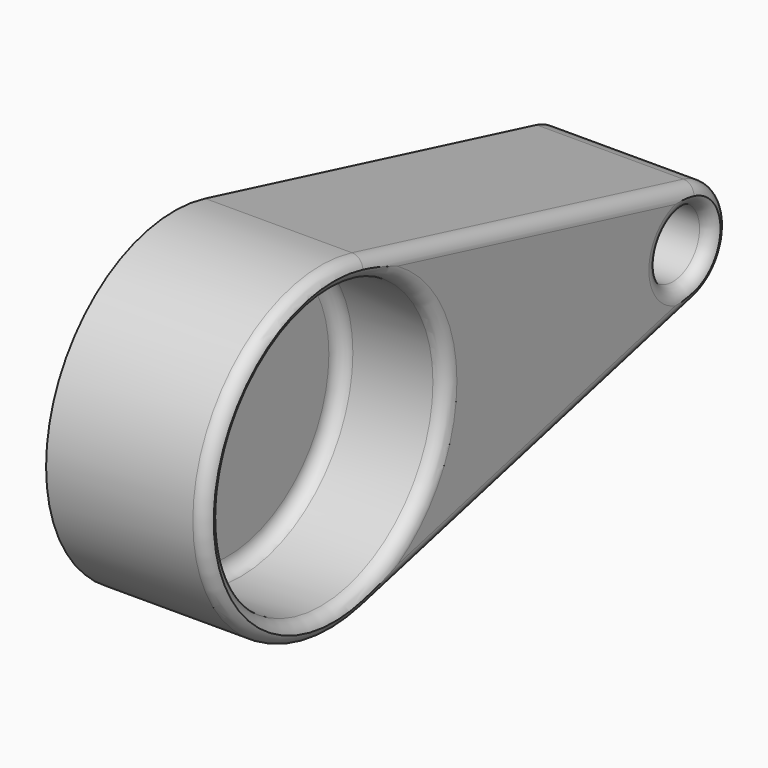
from build123d import *

# Parameters (mm, degrees)
F1_DEPTH = 76.2
F2_R     = 66.675
F2_R_2   = 15.875
F3_DEPTH = 50.8
F4_F1_R  = 6.35
F4_F2_R  = 6.35
F4_F3_R  = 6.35
F5_T     = -2.54


# Not quite as in the source:
# - a fillet or chamfer that OpenCascade refuses, or shapes differently, is made with other operations: its cross-section is extruded or revolved along the edge and cut away or added


with BuildPart() as f1:
    # F0 (on Right) → F1 (new body)
    with BuildSketch(Plane.YZ):
        with BuildLine():
            ThreePointArc((18.4812146278, -73.9248585111), (60.0612543768, -46.8944103565), (76.2, 0))
            ThreePointArc((76.2, 0), (60.0612543768, 46.8944103565), (18.4812146278, 73.9248585111))
            ThreePointArc((18.4812146278, 73.9248585111), (-76.2, 0), (18.4812146278, -73.9248585111))
        make_face()
        with BuildLine():
            ThreePointArc((18.4812146278, 73.9248585111), (60.0612543768, 46.8944103565), (76.2, 0))
            ThreePointArc((76.2, 0), (60.0612543768, -46.8944103565), (18.4812146278, -73.9248585111))
            Line((18.4812146278, -73.9248585111), (215.6141706573, -24.6416195037))
            ThreePointArc((215.6141706573, -24.6416195037), (184.0537657814, 0), (215.6141706573, 24.6416195037))
            Line((215.6141706573, 24.6416195037), (18.4812146278, 73.9248585111))
        make_face()
        with BuildLine():
            ThreePointArc((234.8537657814, 0), (229.474183907, 15.6314701188), (215.6141706573, 24.6416195037))
            ThreePointArc((215.6141706573, 24.6416195037), (184.0537657814, 0), (215.6141706573, -24.6416195037))
            ThreePointArc((215.6141706573, -24.6416195037), (229.474183907, -15.6314701188), (234.8537657814, 0))
        make_face()
    extrude(amount=F1_DEPTH)

    # F2 (on face) → F3 (cut)
    with BuildSketch(Plane.YZ.offset(76.2)):
        Circle(F2_R)
        with Locations((209.4537657814, 0)):
            Circle(F2_R_2)
    extrude(amount=-F3_DEPTH, mode=Mode.SUBTRACT)

    # F4: fillet of radius 6.35 on 8 edges, made by hand

    # F4_f1
    f4_f1_edges = [f1.edges().sort_by_distance(p)[0] for p in [
        (76.2, -76.2, 0),
        (76.2, 117.0476926425, 49.2832390074),
        (76.2, 117.0476926425, -49.2832390074),
        (76.2, 234.8537657814, 0),
    ]]
    fillet(f4_f1_edges, radius=F4_F1_R)

    # F4_f2
    f4_f2_edges = [f1.edges().sort_by_distance(p)[0] for p in [
        (25.4, -66.675, 0),
    ]]
    fillet(f4_f2_edges, radius=F4_F2_R)

    # F4_f3
    f4_f3_edges = [f1.edges().sort_by_distance(p)[0] for p in [
        (25.4, 193.5787657814, 0),
    ]]
    fillet(f4_f3_edges, radius=F4_F3_R)

    # F4_s4 → F4_t5 (revolve, cut)
    with BuildSketch(Plane.XY):
        with BuildLine():
            ThreePointArc((76.2, 73.025), (74.3401280605, 68.5348719395), (69.85, 66.675))
            Line((69.85, 66.675), (69.85, 66.548))
            Line((69.85, 66.548), (76.327, 66.548))
            Line((76.327, 66.548), (76.327, 73.025))
            Line((76.327, 73.025), (76.2, 73.025))
        make_face()
    revolve(axis=Axis((76.2, 0, 0), (1, 0, 0)), mode=Mode.SUBTRACT)

    # F4_s6 → F4_t7 (revolve, cut)
    with BuildSketch(Plane.XY):
        with BuildLine():
            ThreePointArc((69.85, 225.3287657814), (74.3401280605, 227.1886377208), (76.2, 231.6787657814))
            Line((76.2, 231.6787657814), (76.327, 231.6787657814))
            Line((76.327, 231.6787657814), (76.327, 225.2017657814))
            Line((76.327, 225.2017657814), (69.85, 225.2017657814))
            Line((69.85, 225.2017657814), (69.85, 225.3287657814))
        make_face()
    revolve(axis=Axis((76.2, 209.4537657814, 0), (1, 0, 0)), mode=Mode.SUBTRACT)

    # F5
    f5_openings = [f1.faces().sort_by_distance(p)[0] for p in [
        (0, 57.51924, 0),
    ]]
    offset(amount=F5_T, openings=f5_openings)


solid = f1.part
